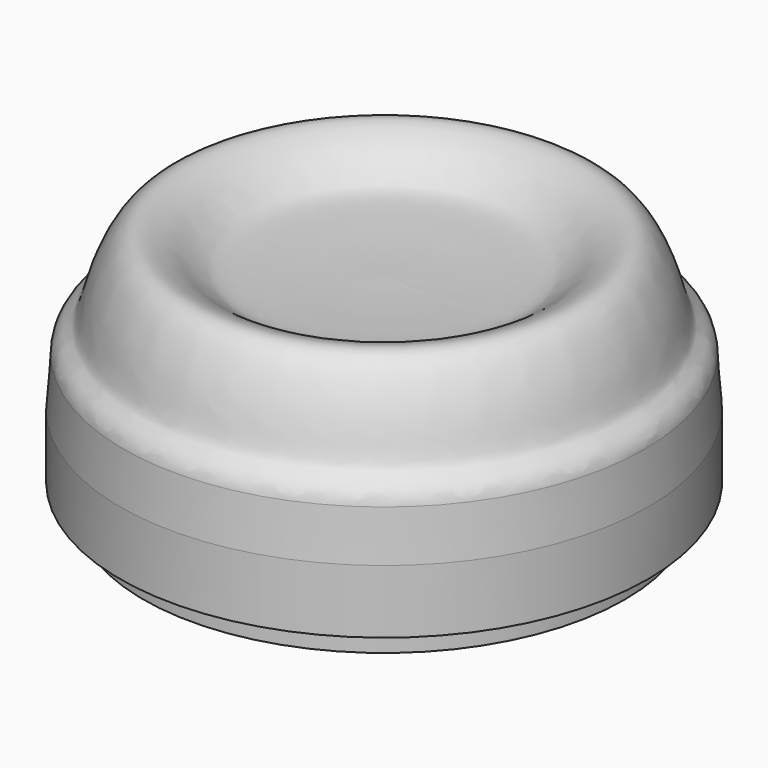
from build123d import *


with BuildPart() as f1:
    # F0 (on Front) → F1 (revolve)
    with BuildSketch(Plane.XZ):
        with BuildLine():
            Line((0, 72.0053985715), (0, 0))
            Line((0, 0), (60.4805797338, 0))
            Line((60.4805797338, 0), (60.4805797338, 2.2335746326))
            Line((60.4805797338, 2.2335746326), (77.0699828863, 6.2070856802))
            Line((77.0699828863, 6.2070856802), (77.0699828863, 14.3860364848))
            Line((77.0699828863, 14.3860364848), (84.5, 14.3860364848))
            Line((84.5, 14.3860364848), (84.5, 34.7170196474))
            Line((84.5, 34.7170196474), (83.3781063557, 50.6331585348))
            add(Edge.make_bspline(
                [(0, 72.0053985715), (5.3624783169, 71.9092158768), (16.3070110762, 71.7129166497), (34.6731579332, 73.0800545991), (43.6552311193, 73.1645561389), (52.6980338602, 81.305037743), (57.0912268293, 83.4401429499), (62.866659385, 85.6198608303), (69.5488472767, 81.1195946469), (75.1692218019, 67.5121489578), (76.8121350319, 58.3757299789), (80.3315916954, 56.4324627805), (83.1774026155, 53.498275578), (83.3781063557, 50.6331585348)],
                knots=[0, 0, 0, 0, 0.1230403877, 0.2511187559, 0.3413960041, 0.4424844079, 0.5106651004, 0.5801720432, 0.6602618119, 0.7773084872, 0.8667002588, 0.923122047, 1, 1, 1, 1], degree=3))
        make_face()
    revolve(axis=Axis((0, 0, 36.0026992857), (0, 0, 1)))


solid = f1.part
